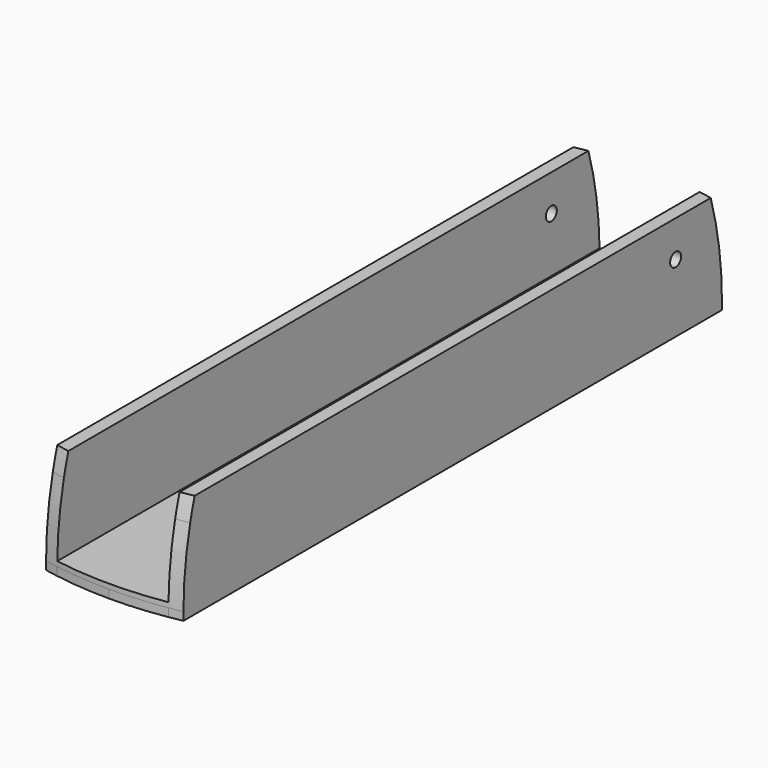
from build123d import *

# Parameters (mm, degrees)
F1_DEPTH      = 4.76
F4_DEPTH      = 38
F8_R          = 2.5
F9_DEPTH      = 4.7610001
F9_DEPTH_BACK = 45.2410001


# Not quite as in the source:
# - a feature names something its author has since deleted; it is built from what else it names


with BuildPart() as f1:
    # F0 (on Top) → F1 (new body)
    with BuildSketch(Plane.XY):
        with BuildLine():
            Line((20.24, 120.3093612318), (20.24, 123.3504860144))
            ThreePointArc((20.24, 123.3504860144), (10.1535522896, 124.5869390261), (0, 125))
            Line((0, 125), (0, 122))
            ThreePointArc((0, 122), (10.1552432202, 121.5766056244), (20.24, 120.3093612318))
        make_face()
        with BuildLine():
            Line((25, 90.3494910666), (25, 119.4110547646))
            ThreePointArc((25, 119.4110547646), (22.6244588582, 119.8838348626), (20.24, 120.3093612318))
            Line((20.24, 120.3093612318), (20.24, 105.3494910666))
            Line((20.24, 105.3494910666), (20.24, 90.3494910666))
            Line((20.24, 90.3494910666), (25, 90.3494910666))
        make_face()
        with BuildLine():
            ThreePointArc((-20.24, -120.3093612318), (-10.1552432202, -121.5766056244), (0, -122))
            Line((0, -122), (0, 0))
            Line((0, 0), (0, 101.8494910666))
            Line((0, 101.8494910666), (-3.5, 101.8494910666))
            Line((-3.5, 101.8494910666), (-3.5, 108.8494910666))
            Line((-3.5, 108.8494910666), (0, 108.8494910666))
            Line((0, 108.8494910666), (0, 122))
            ThreePointArc((0, 122), (-10.1552432202, 121.5766056244), (-20.24, 120.3093612318))
            Line((-20.24, 120.3093612318), (-20.24, 107.6747455333))
            Line((-20.24, 107.6747455333), (-20.24, 90.3494910666))
            Line((-20.24, 90.3494910666), (-20.24, -120.3093612318))
        make_face()
        with BuildLine():
            Line((0, 0), (0, -122))
            ThreePointArc((0, -122), (10.1552432202, -121.5766056244), (20.24, -120.3093612318))
            Line((20.24, -120.3093612318), (20.24, 90.3494910666))
            Line((20.24, 90.3494910666), (20.24, 105.3494910666))
            Line((20.24, 105.3494910666), (20.24, 120.3093612318))
            ThreePointArc((20.24, 120.3093612318), (10.1552432202, 121.5766056244), (0, 122))
            Line((0, 122), (0, 108.8494910666))
            Line((0, 108.8494910666), (3.5, 108.8494910666))
            Line((3.5, 108.8494910666), (3.5, 101.8494910666))
            Line((3.5, 101.8494910666), (0, 101.8494910666))
            Line((0, 101.8494910666), (0, 0))
        make_face()
        with BuildLine():
            Line((0, 122), (0, 125))
            ThreePointArc((0, 125), (-10.1535522896, 124.5869390261), (-20.24, 123.3504860144))
            Line((-20.24, 123.3504860144), (-20.24, 120.3093612318))
            ThreePointArc((-20.24, 120.3093612318), (-10.1552432202, 121.5766056244), (0, 122))
        make_face()
        with BuildLine():
            Line((25, -119.4110547646), (25, 90.3494910666))
            Line((25, 90.3494910666), (20.24, 90.3494910666))
            Line((20.24, 90.3494910666), (20.24, -120.3093612318))
            ThreePointArc((20.24, -120.3093612318), (22.6244588582, -119.8838348626), (25, -119.4110547646))
        make_face()
        with BuildLine():
            ThreePointArc((-20.24, 120.3093612318), (-22.6244588582, 119.8838348626), (-25, 119.4110547646))
            Line((-25, 119.4110547646), (-25, 90.3494910666))
            Line((-25, 90.3494910666), (-20.24, 90.3494910666))
            Line((-20.24, 90.3494910666), (-20.24, 107.6747455333))
            Line((-20.24, 107.6747455333), (-20.24, 120.3093612318))
        make_face()
        with BuildLine():
            ThreePointArc((-25, -119.4110547646), (-22.6244588582, -119.8838348626), (-20.24, -120.3093612318))
            Line((-20.24, -120.3093612318), (-20.24, 90.3494910666))
            Line((-20.24, 90.3494910666), (-25, 90.3494910666))
            Line((-25, 90.3494910666), (-25, -119.4110547646))
        make_face()
    extrude(amount=F1_DEPTH)

    # F0 (on Top) → F4 (join)
    with BuildSketch(Plane.XY):
        with BuildLine():
            ThreePointArc((-20.24, 123.3504860144), (-22.6242401752, 122.9355268281), (-25, 122.4744871392))
            Line((-25, 122.4744871392), (-25, 119.4110547646))
            ThreePointArc((-25, 119.4110547646), (-22.6244588582, 119.8838348626), (-20.24, 120.3093612318))
            Line((-20.24, 120.3093612318), (-20.24, 123.3504860144))
        make_face()
        with BuildLine():
            ThreePointArc((-20.24, 120.3093612318), (-22.6244588582, 119.8838348626), (-25, 119.4110547646))
            Line((-25, 119.4110547646), (-25, 90.3494910666))
            Line((-25, 90.3494910666), (-20.24, 90.3494910666))
            Line((-20.24, 90.3494910666), (-20.24, 107.6747455333))
            Line((-20.24, 107.6747455333), (-20.24, 120.3093612318))
        make_face()
        with BuildLine():
            Line((25, 90.3494910666), (25, 119.4110547646))
            ThreePointArc((25, 119.4110547646), (22.6244588582, 119.8838348626), (20.24, 120.3093612318))
            Line((20.24, 120.3093612318), (20.24, 105.3494910666))
            Line((20.24, 105.3494910666), (20.24, 90.3494910666))
            Line((20.24, 90.3494910666), (25, 90.3494910666))
        make_face()
        with BuildLine():
            Line((25, 119.4110547646), (25, 122.4744871392))
            ThreePointArc((25, 122.4744871392), (22.6242401752, 122.9355268281), (20.24, 123.3504860144))
            Line((20.24, 123.3504860144), (20.24, 120.3093612318))
            ThreePointArc((20.24, 120.3093612318), (22.6244588582, 119.8838348626), (25, 119.4110547646))
        make_face()
        with BuildLine():
            Line((25, -119.4110547646), (25, 90.3494910666))
            Line((25, 90.3494910666), (20.24, 90.3494910666))
            Line((20.24, 90.3494910666), (20.24, -120.3093612318))
            ThreePointArc((20.24, -120.3093612318), (22.6244588582, -119.8838348626), (25, -119.4110547646))
        make_face()
        with BuildLine():
            ThreePointArc((-25, -119.4110547646), (-22.6244588582, -119.8838348626), (-20.24, -120.3093612318))
            Line((-20.24, -120.3093612318), (-20.24, 90.3494910666))
            Line((-20.24, 90.3494910666), (-25, 90.3494910666))
            Line((-25, 90.3494910666), (-25, -119.4110547646))
        make_face()
    extrude(amount=F4_DEPTH)

    # F2 (on Front) → F6 (revolve, cut)
    with BuildSketch(Plane.XZ):
        with BuildLine():
            ThreePointArc((0, 128), (88.3883476483, 91.3883476483), (125, 3))
            Line((125, 3), (150, 3))
            ThreePointArc((150, 3), (106.066017178, 109.066017178), (0, 153))
            Line((0, 153), (0, 128))
        make_face()
    revolve(axis=Axis((0, 0, 64), (0, 0, 1)), mode=Mode.SUBTRACT)

    # F7: F1 across face


with BuildPart() as f1_1:
    add(f1.part)
    add(f1.part.mirror(Plane.XZ))

    # F8 (on face) → F9 (cut, two sides)
    with BuildSketch(Plane(origin=(20.24, 0, 0), x_dir=(0, -1, 0), z_dir=(-1, 0, 0))) as f9_sk:
        with Locations((-101.4159989458, 24.76)):
            Circle(F8_R)
    extrude(amount=-F9_DEPTH, mode=Mode.SUBTRACT)
    extrude(f9_sk.sketch, amount=F9_DEPTH_BACK, mode=Mode.SUBTRACT)


solid = f1_1.part
